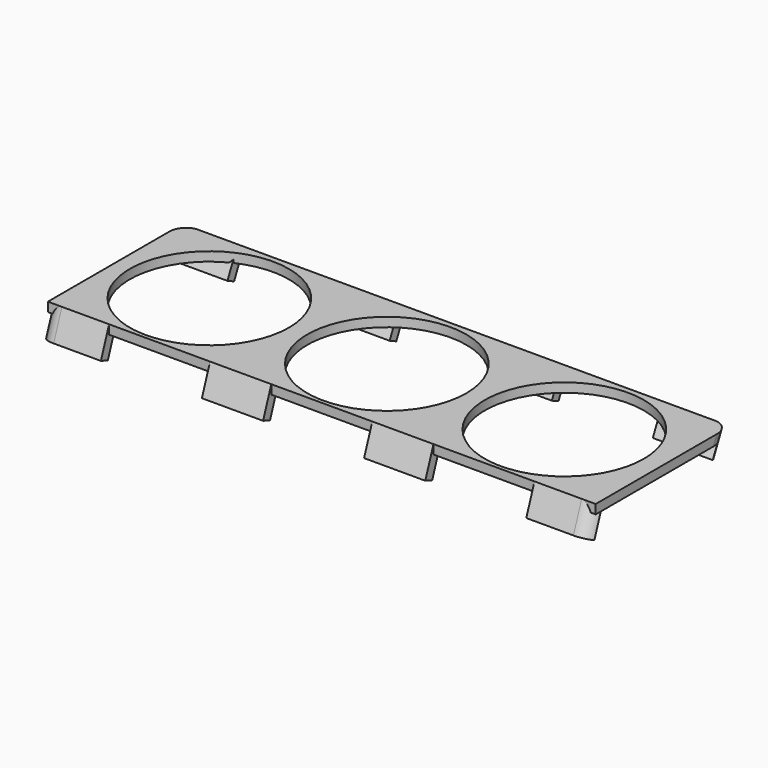
from build123d import *

# Parameters (mm, degrees)
F0_W           = 179
F0_H           = 55
F0_R           = 26
F1_DEPTH       = 3
F7_DEPTH       = 179.001
F8_W           = 20
F8_H           = 6
F9_DEPTH       = 3
F10_W          = 20
F10_H          = 9.7746569663
F11_DEPTH      = 3
F12_F1_R       = 5
F12_F2_R       = 5
F12_2_T1_DEPTH = 32.6875354411
F12_3_T1_DEPTH = 32.6875354411


# Not quite as in the source:
# - a fillet or chamfer that OpenCascade refuses, or shapes differently, is made with other operations: its cross-section is extruded or revolved along the edge and cut away or added


with BuildPart() as f1:
    # F0 (on Top) → F1 (new body)
    with BuildSketch(Plane.XY):
        with Locations((-89.5, 27.5)):
            Rectangle(F0_W, F0_H)
        with Locations((-148, 27.2)):
            Circle(F0_R, mode=Mode.SUBTRACT)
        with Locations((-90, 27.2)):
            Circle(F0_R, mode=Mode.SUBTRACT)
        with Locations((-32, 27.2)):
            Circle(F0_R, mode=Mode.SUBTRACT)
    extrude(amount=-F1_DEPTH)

    # F6 (on offset) → F7 (cut, through all)
    with BuildSketch(Plane(origin=(-179, 0, 0), x_dir=(0, -1, 0), z_dir=(-1, 0, 0))):
        Polygon((-49.9016099183, -10.9335328137), (-55, 0), (-57.2723100997, -1.0595956012), (-52.2457129351, -11.8391680074), align=None)
    extrude(amount=-F7_DEPTH, mode=Mode.SUBTRACT)

    # F8 (on face) → F9 (join)
    with BuildSketch(Plane(origin=(0, 45.1766592664, -21.0662221858), x_dir=(1, 0, 0), z_dir=(0, -0.906307787, 0.4226182617))):
        with Locations((-10, 16.9338706389)):
            Rectangle(F8_W, F8_H)
        with Locations((-169, 16.9338706389)):
            Rectangle(F8_W, F8_H)
        with Locations((-116, 16.9338706389)):
            Rectangle(F8_W, F8_H)
        with Locations((-63, 16.9338706389)):
            Rectangle(F8_W, F8_H)
    extrude(amount=F9_DEPTH)

    # F12: fillet of radius 5 on 2 edges, made by hand

    # F12_f1
    f12_f1_edges = [f1.edges().sort_by_distance(p)[0] for p in [
        (-179, 53.0326837275, -4.2189233611),
    ]]
    fillet(f12_f1_edges, radius=F12_F1_R)

    # F12_f2
    f12_f2_edges = [f1.edges().sort_by_distance(p)[0] for p in [
        (0, 53.0326837275, -4.2189233611),
    ]]
    fillet(f12_f2_edges, radius=F12_F2_R)


with BuildPart() as f11:
    # F10 (on face) → F11 (new body)
    with BuildSketch(Plane(origin=(0, 0, 0), x_dir=(1, 0, 0), z_dir=(0, -0.9396926208, 0.3420201433))):
        with Locations((-10, -4.8873284832)):
            Rectangle(F10_W, F10_H)
    extrude(amount=-F11_DEPTH)

    # F12#2: fillet of radius 5 on 1 edges, made by hand

    # F12_2_s2 → F12_2_t1 (cut)
    with BuildSketch(Plane(origin=(0, -7.2614625666, -19.9507044338), x_dir=(1, 0, 0), z_dir=(0, 0.3420201433, 0.9396926208))):
        with BuildLine():
            ThreePointArc((0, 3), (-1.8439629074, 0.8166998673), (-4.582575695, 0))
            Line((-4.582575695, 0), (0, 0))
            Line((0, 0), (0, 3))
        make_face()
    extrude(amount=F12_2_T1_DEPTH, mode=Mode.SUBTRACT)


with BuildPart() as f11b:
    # F10 (on face) → F11, piece 2 (new body)
    with BuildSketch(Plane(origin=(0, 0, 0), x_dir=(1, 0, 0), z_dir=(0, -0.9396926208, 0.3420201433))):
        with Locations((-169, -4.8873284832)):
            Rectangle(F10_W, F10_H)
    extrude(amount=-F11_DEPTH)

    # F12#3: fillet of radius 5 on 1 edges, made by hand

    # F12_3_s2 → F12_3_t1 (cut)
    with BuildSketch(Plane(origin=(0, 3.91833299, 10.7655314119), x_dir=(1, 0, 0), z_dir=(0, -0.3420201433, -0.9396926208))):
        with BuildLine():
            ThreePointArc((-179, -3), (-177.1560370926, -0.8166998673), (-174.417424305, 0))
            Line((-174.417424305, 0), (-179, 0))
            Line((-179, 0), (-179, -3))
        make_face()
    extrude(amount=F12_3_T1_DEPTH, mode=Mode.SUBTRACT)


with BuildPart() as f11c:
    # F10 (on face) → F11, piece 3 (new body)
    with BuildSketch(Plane(origin=(0, 0, 0), x_dir=(1, 0, 0), z_dir=(0, -0.9396926208, 0.3420201433))):
        with Locations((-116, -4.8873284832)):
            Rectangle(F10_W, F10_H)
    extrude(amount=-F11_DEPTH)


with BuildPart() as f11d:
    # F10 (on face) → F11, piece 4 (new body)
    with BuildSketch(Plane(origin=(0, 0, 0), x_dir=(1, 0, 0), z_dir=(0, -0.9396926208, 0.3420201433))):
        with Locations((-63, -4.8873284832)):
            Rectangle(F10_W, F10_H)
    extrude(amount=-F11_DEPTH)


solid = Compound([f1.part, f11.part, f11b.part, f11c.part, f11d.part])
